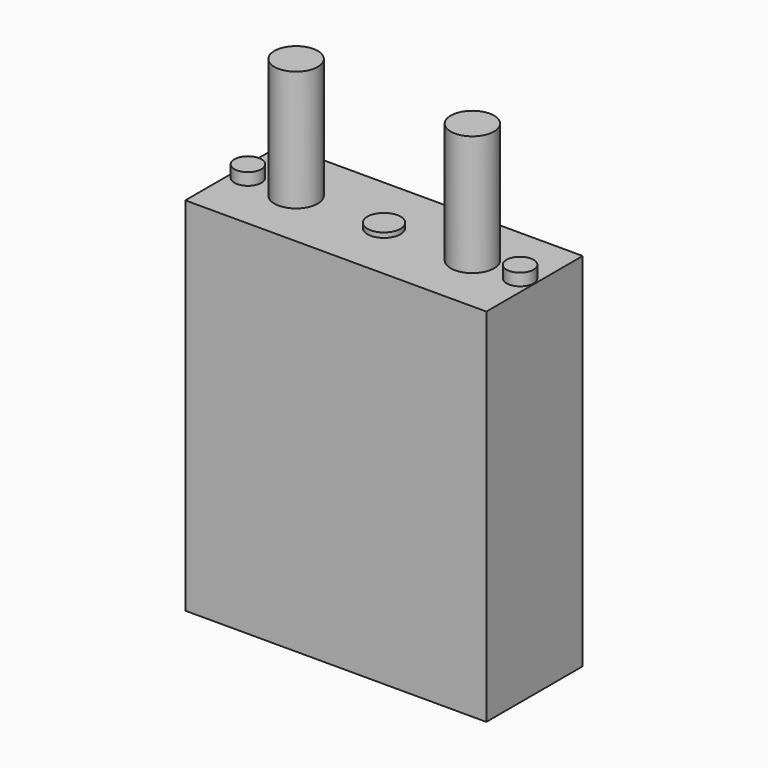
from build123d import *

# Parameters (mm, degrees)
F0_W     = 31.75
F0_H     = 6.35
F1_DEPTH = 12.7
F2_R     = 1.4204821808
F3_DEPTH = 1.27
F2_R_2   = 1.7458442661
F4_DEPTH = 0.508
F2_R_3   = 2.2844516469
F6_DEPTH = 12.7


# Not quite as in the source:
# - the program builds the solid bodies; features that only make, move or delete a surface that nothing else refers to are left out


with BuildPart() as f1:
    # F0 (on Front) → F1 (new body)
    with BuildSketch(Plane.XZ):
        with Locations((0, 15.875)):
            Rectangle(F0_W, F0_H)
        with Locations((0, 9.525)):
            Rectangle(F0_W, F0_H)
        with Locations((0, 3.175)):
            Rectangle(F0_W, F0_H)
        with Locations((0, -3.175)):
            Rectangle(F0_W, F0_H)
        with Locations((0, -9.525)):
            Rectangle(F0_W, F0_H)
        with Locations((0, -15.875)):
            Rectangle(F0_W, F0_H)
    extrude(amount=-F1_DEPTH)

    # F2 (on face) → F3 (join)
    with BuildSketch(Plane.XY.offset(19.05)):
        with Locations((-14.351, 6.35)):
            Circle(F2_R)
        with Locations((14.351, 6.35)):
            Circle(F2_R)
    extrude(amount=F3_DEPTH)

    # F2 (on face) → F4 (join)
    with BuildSketch(Plane.XY.offset(19.05)):
        with Locations((0, 6.35)):
            Circle(F2_R_2)
    extrude(amount=F4_DEPTH)

    # F2 (on face) → F6 (join)
    with BuildSketch(Plane.XY.offset(19.05)):
        with Locations((-9.271, 6.35)):
            Circle(F2_R_3)
        with Locations((9.271, 6.4142975025)):
            Circle(F2_R_3)
    extrude(amount=F6_DEPTH)


solid = f1.part
